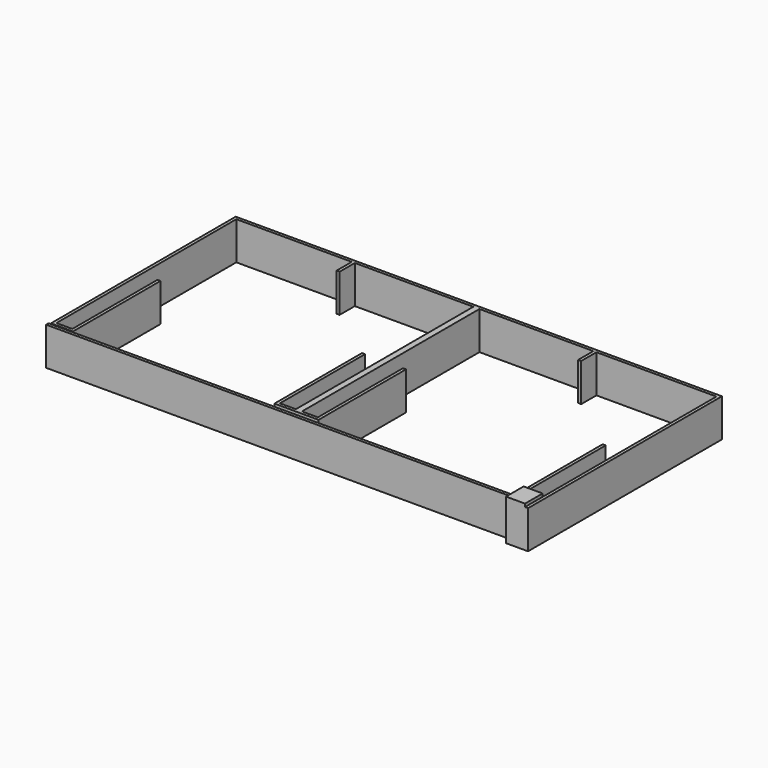
from build123d import *

# Parameters (mm, degrees)
F0_W      = 640
F0_H      = 50
F1_DEPTH  = 4
F2_W      = 4
F2_H      = 50
F3_DEPTH  = 300
F4_W      = 4
F4_H      = 50
F5_DEPTH  = 300
F6_W      = 4
F6_H      = 50
F7_DEPTH  = 25
F8_W      = 4
F8_H      = 50
F9_DEPTH  = 25
F10_W     = 8
F10_H     = 50
F11_DEPTH = 300
F12_W     = 4
F12_H     = 50
F13_DEPTH = 25
F14_W     = 4
F14_H     = 50
F15_DEPTH = 25
F16_W     = 4
F16_H     = 50
F17_DEPTH = 140
F18_W     = 4
F18_H     = 50
F19_DEPTH = 140
F22_W     = 4
F22_H     = 50
F23_DEPTH = 25
F24_W     = 4
F24_H     = 50
F25_DEPTH = 140
F26_W     = 4
F26_H     = 50
F27_DEPTH = 140
F28_W     = 4
F28_H     = 25
F29_DEPTH = 50
F31_W     = 4
F31_H     = 50
F32_DEPTH = 15
F33_W     = 4
F33_H     = 50
F34_DEPTH = 25
F35_W     = 25
F35_H     = 4
F36_DEPTH = 4
F37_W     = 25
F37_H     = 3.9
F38_DEPTH = 25
F39_W     = 4
F39_H     = 50
F40_DEPTH = 638


# Not quite as in the source:
# - a feature of the source that left no trace in its solid (it failed there, or was rolled back) is left out
# - the program builds the solid bodies; features that only make, move or delete a surface that nothing else refers to are left out


with BuildPart() as f1:
    # F0 (on Front) → F1 (new body)
    with BuildSketch(Plane.XZ):
        Rectangle(F0_W, F0_H)
    extrude(amount=F1_DEPTH)

    # F2 (on face) → F3 (join)
    with BuildSketch(Plane.XZ.offset(4)):
        with Locations((-318, 0)):
            Rectangle(F2_W, F2_H)
    extrude(amount=F3_DEPTH)

    # F4 (on face) → F5 (join)
    with BuildSketch(Plane.XZ.offset(4)):
        with Locations((318, 0)):
            Rectangle(F4_W, F4_H)
    extrude(amount=F5_DEPTH)

    # F6 (on face) → F7 (join)
    with BuildSketch(Plane.YZ.offset(-316)):
        with Locations((-302, 0)):
            Rectangle(F6_W, F6_H)
    extrude(amount=F7_DEPTH)

    # F8 (on face) → F9 (join)
    with BuildSketch(Plane(origin=(316, 0, 0), x_dir=(0, -1, 0), z_dir=(-1, 0, 0))):
        with Locations((302, 0)):
            Rectangle(F8_W, F8_H)
    extrude(amount=F9_DEPTH)

    # F10 (on Front) → F11 (join)
    with BuildSketch(Plane.XZ):
        Rectangle(F10_W, F10_H)
    extrude(amount=F11_DEPTH)

    # F12 (on face) → F13 (join)
    with BuildSketch(Plane.XZ.offset(4)):
        with Locations((-162, 0)):
            Rectangle(F12_W, F12_H)
    extrude(amount=F13_DEPTH)

    # F14 (on face) → F15 (join)
    with BuildSketch(Plane(origin=(-4, 0, 0), x_dir=(0, -1, 0), z_dir=(-1, 0, 0))):
        with Locations((298, 0)):
            Rectangle(F14_W, F14_H)
    extrude(amount=F15_DEPTH)

    # F16 (on face) → F17 (join)
    with BuildSketch(Plane(origin=(0, -300, 0), x_dir=(-1, 0, 0), z_dir=(0, 1, 0))):
        with Locations((293, 0)):
            Rectangle(F16_W, F16_H)
    extrude(amount=F17_DEPTH)

    # F18 (on face) → F19 (join)
    with BuildSketch(Plane(origin=(0, -296, 0), x_dir=(-1, 0, 0), z_dir=(0, 1, 0))):
        with Locations((27, 0)):
            Rectangle(F18_W, F18_H)
    extrude(amount=F19_DEPTH)

    # F22 (on face) → F23 (join)
    with BuildSketch(Plane.YZ.offset(4)):
        with Locations((-298, 0)):
            Rectangle(F22_W, F22_H)
    extrude(amount=F23_DEPTH)

    # F24 (on face) → F25 (join)
    with BuildSketch(Plane(origin=(0, -296, 0), x_dir=(-1, 0, 0), z_dir=(0, 1, 0))):
        with Locations((-27, 0)):
            Rectangle(F24_W, F24_H)
    extrude(amount=F25_DEPTH)

    # F26 (on face) → F27 (join)
    with BuildSketch(Plane(origin=(0, -300, 0), x_dir=(-1, 0, 0), z_dir=(0, 1, 0))):
        with Locations((-293, 0)):
            Rectangle(F26_W, F26_H)
    extrude(amount=F27_DEPTH)

    # F31 (on face) → F32 (join)
    with BuildSketch(Plane.XZ.offset(304)):
        with Locations((318, 0)):
            Rectangle(F31_W, F31_H)
    extrude(amount=F32_DEPTH)

    # F33 (on face) → F34 (join)
    with BuildSketch(Plane(origin=(316, 0, 0), x_dir=(0, -1, 0), z_dir=(-1, 0, 0))):
        with Locations((317, 0)):
            Rectangle(F33_W, F33_H)
    extrude(amount=F34_DEPTH)

    # F35 (on face) → F36 (join)
    with BuildSketch(Plane.XY.offset(25)):
        with Locations((303.5, -317)):
            Rectangle(F35_W, F35_H)
    extrude(amount=F36_DEPTH)

    # F37 (on face) → F38 (join)
    with BuildSketch(Plane(origin=(0, -315, 0), x_dir=(-1, 0, 0), z_dir=(0, 1, 0))):
        with Locations((-303.5, 27.05)):
            Rectangle(F37_W, F37_H)
    extrude(amount=F38_DEPTH)

    # F39 (on face) → F40 (join)
    with BuildSketch(Plane(origin=(316, 0, 0), x_dir=(0, -1, 0), z_dir=(-1, 0, 0))):
        with Locations((307.5, 0)):
            Rectangle(F39_W, F39_H)
    extrude(amount=F40_DEPTH)


with BuildPart() as f29:
    # F28 (on face) → F29 (new body)
    with BuildSketch(Plane(origin=(0, 0, -25), x_dir=(1, 0, 0), z_dir=(0, 0, -1))):
        with Locations((156, 16.5)):
            Rectangle(F28_W, F28_H)
    extrude(amount=-F29_DEPTH)


solid = Compound([f1.part, f29.part])
